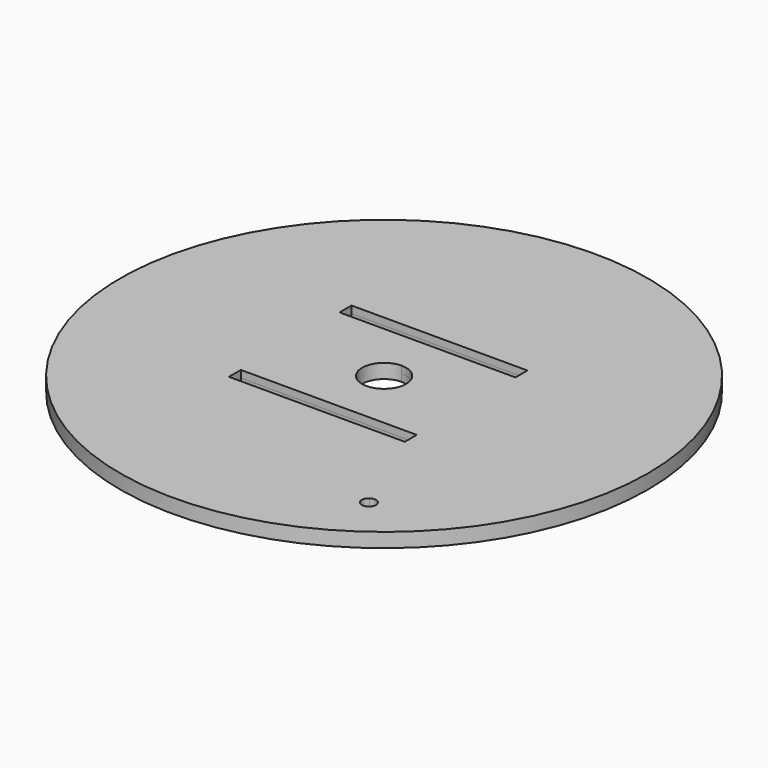
from build123d import *

# Parameters (mm, degrees)
F1_DEPTH = 1.625


# Not quite as in the source:
# - a feature names something its author has since deleted; it is built from what else it names


with BuildPart() as f1:
    # F0 (on Top) → F1 (new body, symmetric)
    with BuildSketch(Plane.XY):
        with BuildLine():
            ThreePointArc((-0.2115118035, -59.9996271885), (42.3515601353, -42.5011217982), (60, 0))
            ThreePointArc((60, 0), (-42.3515601353, 42.5011217982), (-0.2115118035, -59.9996271885))
        make_face()
        with BuildLine():
            ThreePointArc((29.8884344963, -39.6833022032), (28.7759960304, -41.2072063178), (26.9855798083, -40.6120484882))
            ThreePointArc((26.9855798083, -40.6120484882), (26.7104543153, -39.4187676146), (27.3596882112, -38.3804475152))
            ThreePointArc((27.3596882112, -38.3804475152), (29.0212393625, -38.2609812028), (29.8884344963, -39.6833022032))
        make_face(mode=Mode.SUBTRACT)
        with BuildLine():
            Line((18.7182445079, -17.5), (12.4749599, -17.5))
            Line((12.4749599, -17.5), (0, -17.5))
            Line((0, -17.5), (-21.2817554921, -17.5))
            Line((-21.2817554921, -17.5), (-21.2817554921, -14.1))
            Line((-21.2817554921, -14.1), (-11.0323727131, -14.1))
            Line((-11.0323727131, -14.1), (-11.0323727131, 14.1))
            Line((-11.0323727131, 14.1), (-21.4130617678, 14.1))
            Line((-21.4130617678, 14.1), (-21.4130617678, 17.5))
            Line((-21.4130617678, 17.5), (0, 17.5))
            Line((0, 17.5), (18.5869382322, 17.5))
            Line((18.5869382322, 17.5), (18.5869382322, 14.1))
            Line((18.5869382322, 14.1), (0, 14.1))
            Line((0, 14.1), (0, 5))
            ThreePointArc((0, 5), (3.5355339059, 3.5355339059), (5, 0))
            ThreePointArc((5, 0), (4.4447531261, -2.290015207), (2.9023321408, -4.0714209))
            Line((2.9023321408, -4.0714209), (10.0512534051, -14.1))
            Line((10.0512534051, -14.1), (18.7182445079, -14.1))
            Line((18.7182445079, -14.1), (18.7182445079, -17.5))
        make_face(mode=Mode.SUBTRACT)
        with BuildLine():
            Line((0, -14.1), (10.0512534051, -14.1))
            Line((10.0512534051, -14.1), (2.9023321408, -4.0714209))
            ThreePointArc((2.9023321408, -4.0714209), (1.5236297943, -4.762200358), (0, -5))
            Line((0, -5), (0, -14.1))
        make_face()
        with BuildLine():
            Line((-11.0323727131, -14.1), (0, -14.1))
            Line((0, -14.1), (0, -5))
            ThreePointArc((0, -5), (-5, 0), (0, 5))
            Line((0, 5), (0, 14.1))
            Line((0, 14.1), (-11.0323727131, 14.1))
            Line((-11.0323727131, 14.1), (-11.0323727131, -14.1))
        make_face()
    extrude(amount=F1_DEPTH, both=True)


solid = f1.part
